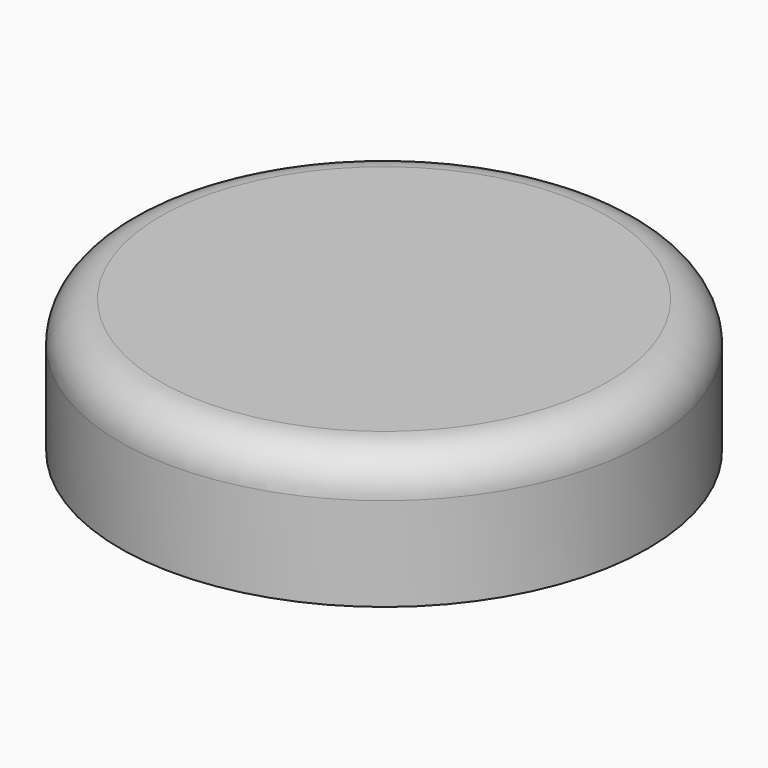
from build123d import *

# Parameters (mm, degrees)
F2_R     = 19.75
F2_R_2   = 17.75
F3_DEPTH = 10
F4_DEPTH = 7
F5_R     = 3


with BuildPart() as f3:
    # F2 (on Top) → F3 (new body)
    with BuildSketch(Plane.XY):
        Circle(F2_R)
        Circle(F2_R_2, mode=Mode.SUBTRACT)
        Circle(F2_R_2)
    extrude(amount=F3_DEPTH)

    # F2 (on Top) → F4 (cut)
    with BuildSketch(Plane.XY):
        Circle(F2_R_2)
    extrude(amount=F4_DEPTH, mode=Mode.SUBTRACT)

    # F5
    f5_edges = [f3.edges().sort_by_distance(p)[0] for p in [
        (-19.75, 0, 10),
    ]]
    fillet(f5_edges, radius=F5_R)


solid = f3.part
